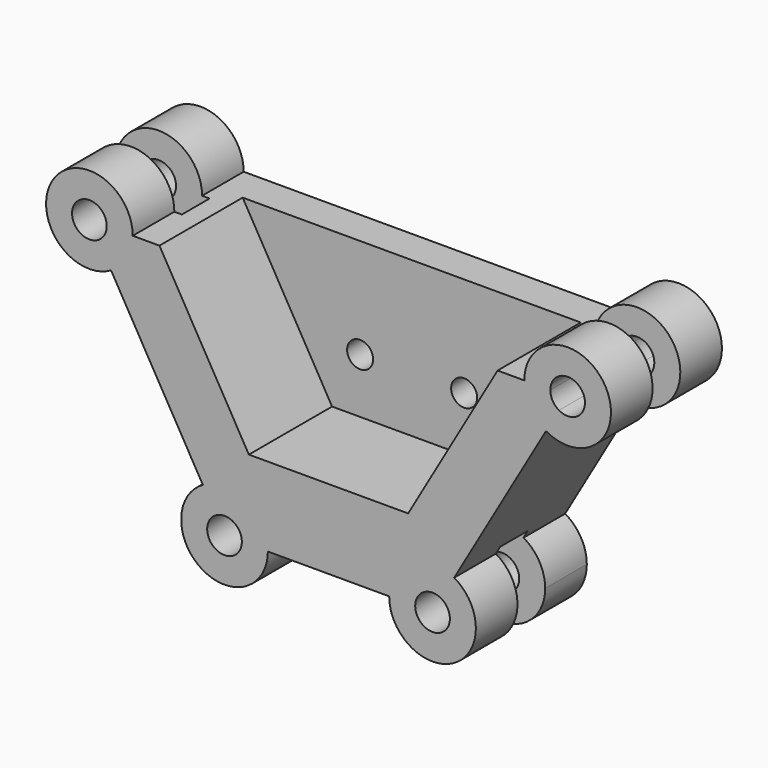
from build123d import *

# Parameters (mm, degrees)
F1_DEPTH = 50.8
F3_DEPTH = 76.2
F4_R     = 38.1
F5_DEPTH = 12.7
F7_R     = 9.525
F8_DEPTH = 50.801


with BuildPart() as f1:
    # F0 (on Front) → F1 (new body, symmetric)
    with BuildSketch(Plane.XZ):
        with BuildLine():
            ThreePointArc((-92.3535701347, -59.3866830272), (-60.6035701347, -59.3866830272), (-44.7285701347, -86.8829895973))
            Line((-44.7285701347, -86.8829895973), (44.1714298653, -86.8829895973))
            ThreePointArc((44.1714298653, -86.8829895973), (60.0464298653, -59.3866830272), (91.7964298653, -59.3866830272))
            Line((91.7964298653, -59.3866830272), (159.0331335179, 57.0707038325))
            ThreePointArc((159.0331335179, 57.0707038325), (147.4118269477, 68.6920104027), (143.1581335179, 84.5670104027))
            Line((143.1581335179, 84.5670104027), (-143.7152737873, 84.5670104027))
            ThreePointArc((-143.7152737873, 84.5670104027), (-147.9689672171, 68.6920104027), (-159.5902737873, 57.0707038325))
            Line((-159.5902737873, 57.0707038325), (-92.3535701347, -59.3866830272))
        make_face()
        with BuildLine():
            ThreePointArc((-143.7152737873, 84.5670104027), (-202.9615803574, 100.4420104027), (-159.5902737873, 57.0707038325))
            Line((-159.5902737873, 57.0707038325), (-169.1152737873, 73.5684877746))
            ThreePointArc((-169.1152737873, 73.5684877746), (-186.4637964153, 90.9170104027), (-162.7652737873, 84.5670104027))
            Line((-162.7652737873, 84.5670104027), (-143.7152737873, 84.5670104027))
        make_face()
        with BuildLine():
            Line((-169.1152737873, 73.5684877746), (-159.5902737873, 57.0707038325))
            ThreePointArc((-159.5902737873, 57.0707038325), (-147.9689672171, 68.6920104027), (-143.7152737873, 84.5670104027))
            Line((-143.7152737873, 84.5670104027), (-162.7652737873, 84.5670104027))
            ThreePointArc((-162.7652737873, 84.5670104027), (-164.4667511592, 78.2170104027), (-169.1152737873, 73.5684877746))
        make_face()
        with BuildLine():
            ThreePointArc((143.1581335179, 84.5670104027), (147.4118269477, 68.6920104027), (159.0331335179, 57.0707038325))
            Line((159.0331335179, 57.0707038325), (168.5581335179, 73.5684877746))
            ThreePointArc((168.5581335179, 73.5684877746), (163.9096108898, 78.2170104027), (162.2081335179, 84.5670104027))
            Line((162.2081335179, 84.5670104027), (143.1581335179, 84.5670104027))
        make_face()
        with BuildLine():
            Line((168.5581335179, 73.5684877746), (159.0331335179, 57.0707038325))
            ThreePointArc((159.0331335179, 57.0707038325), (190.7831335179, 57.0707038325), (206.6581335179, 84.5670104027))
            ThreePointArc((206.6581335179, 84.5670104027), (174.9081335179, 116.3170104027), (143.1581335179, 84.5670104027))
            Line((143.1581335179, 84.5670104027), (162.2081335179, 84.5670104027))
            ThreePointArc((162.2081335179, 84.5670104027), (174.9081335179, 97.2670104027), (187.6081335179, 84.5670104027))
            ThreePointArc((187.6081335179, 84.5670104027), (181.2581335179, 73.5684877746), (168.5581335179, 73.5684877746))
        make_face()
        with BuildLine():
            ThreePointArc((91.7964298653, -59.3866830272), (60.0464298653, -59.3866830272), (44.1714298653, -86.8829895973))
            Line((44.1714298653, -86.8829895973), (63.2214298653, -86.8829895973))
            ThreePointArc((63.2214298653, -86.8829895973), (69.5714298653, -75.8844669693), (82.2714298653, -75.8844669693))
            Line((82.2714298653, -75.8844669693), (91.7964298653, -59.3866830272))
        make_face()
        with BuildLine():
            Line((63.2214298653, -86.8829895973), (44.1714298653, -86.8829895973))
            ThreePointArc((44.1714298653, -86.8829895973), (75.9214298653, -118.6329895973), (107.6714298653, -86.8829895973))
            ThreePointArc((107.6714298653, -86.8829895973), (103.4177364354, -71.0079895973), (91.7964298653, -59.3866830272))
            Line((91.7964298653, -59.3866830272), (82.2714298653, -75.8844669693))
            ThreePointArc((82.2714298653, -75.8844669693), (86.9199524934, -80.5329895973), (88.6214298653, -86.8829895973))
            ThreePointArc((88.6214298653, -86.8829895973), (75.9214298653, -99.5829895973), (63.2214298653, -86.8829895973))
        make_face()
        with BuildLine():
            ThreePointArc((-82.8285701347, -75.8844669693), (-70.1285701347, -75.8844669693), (-63.7785701347, -86.8829895973))
            Line((-63.7785701347, -86.8829895973), (-44.7285701347, -86.8829895973))
            ThreePointArc((-44.7285701347, -86.8829895973), (-60.6035701347, -59.3866830272), (-92.3535701347, -59.3866830272))
            Line((-92.3535701347, -59.3866830272), (-82.8285701347, -75.8844669693))
        make_face()
        with BuildLine():
            Line((-44.7285701347, -86.8829895973), (-63.7785701347, -86.8829895973))
            ThreePointArc((-63.7785701347, -86.8829895973), (-82.8285701347, -97.8815122254), (-82.8285701347, -75.8844669693))
            Line((-82.8285701347, -75.8844669693), (-92.3535701347, -59.3866830272))
            ThreePointArc((-92.3535701347, -59.3866830272), (-92.3535701347, -114.3792961675), (-44.7285701347, -86.8829895973))
        make_face()
    extrude(amount=F1_DEPTH, both=True)

    # F2 (on face) → F3 (cut)
    with BuildSketch(Plane.XZ.offset(50.8)):
        Polygon((123.5816945869, 84.5670104027), (-124.1388348563, 84.5670104027), (-58.6310365333, -28.8958245848), (58.0738962639, -28.8958245848), align=None)
    extrude(amount=-F3_DEPTH, mode=Mode.SUBTRACT)

    # F4 (on Front) → F5 (cut, symmetric)
    with BuildSketch(Plane.XZ):
        with Locations((-176.3127177301, 84.7191157899)):
            Circle(F4_R)
        with Locations((176.0305875596, 85.0320324617)):
            Circle(F4_R)
        with Locations((76.2104084713, -87.0717109253)):
            Circle(F4_R)
        with Locations((-77.118386936, -87.0717109253)):
            Circle(F4_R)
    extrude(amount=F5_DEPTH, both=True, mode=Mode.SUBTRACT)

    # F7 (on face) → F8 (cut, through all)
    with BuildSketch(Plane.XZ):
        with Locations((-38.1, 11.3160433248)):
            Circle(F7_R)
        with Locations((38.1, 11.3160433248)):
            Circle(F7_R)
    extrude(amount=-F8_DEPTH, mode=Mode.SUBTRACT)


solid = f1.part
